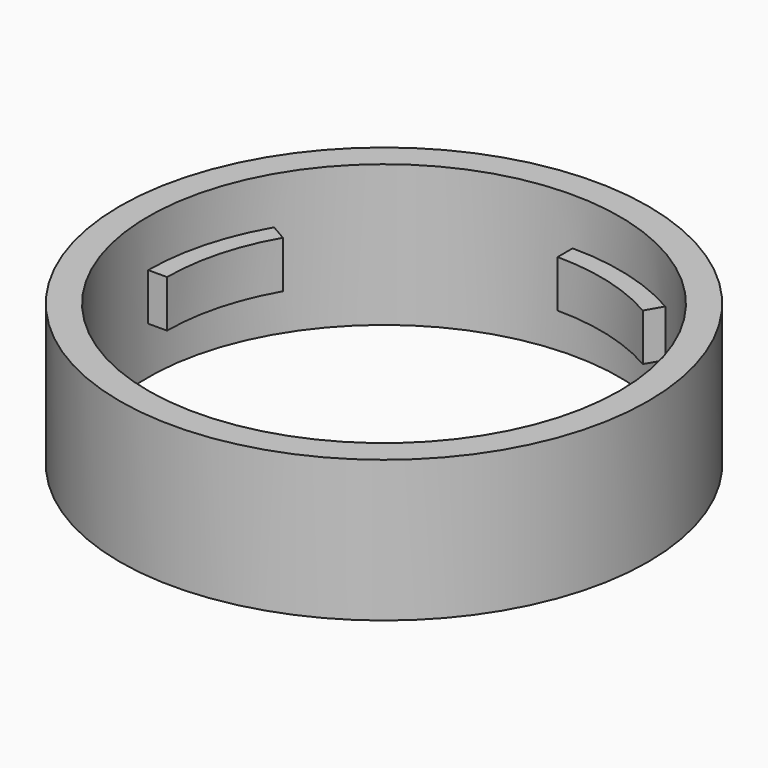
from build123d import *

# Parameters (mm, degrees)
F0_R            = 28
F0_R_2          = 25
F1_DEPTH        = 15
F4_DEPTH        = 2.5
F4_COPIES_COUNT = 4


# Not quite as in the source:
# - a pattern or mirror of a feature is missing from the dataset's text; its kind, count and spacing are read off the source's solid


with BuildPart() as f1:
    # F0 (on Top) → F1 (new body)
    with BuildSketch(Plane.XY):
        Circle(F0_R)
        Circle(F0_R_2, mode=Mode.SUBTRACT)
    extrude(amount=F1_DEPTH)

    # F3 (on offset) → F4 (join, symmetric)
    with BuildSketch(Plane.XY.offset(7.5)):
        with BuildLine():
            ThreePointArc((0, 23), (5.9528380374, 22.2162940046), (11.5, 19.918584287))
            Line((11.5, 19.918584287), (12.5, 21.6506350946))
            ThreePointArc((12.5, 21.6506350946), (6.4704761276, 24.1481456572), (0, 25))
            Line((0, 25), (0, 23))
        make_face()
    f4 = extrude(amount=F4_DEPTH, both=True)

    # F4_copies: F4 ×4 about axis
    f4_copies_axis = Axis((0, 0, 0), (0, 0, 1))
    for i in range(1, F4_COPIES_COUNT):
        add(f4.rotate(f4_copies_axis, i * 360 / F4_COPIES_COUNT))


solid = f1.part
